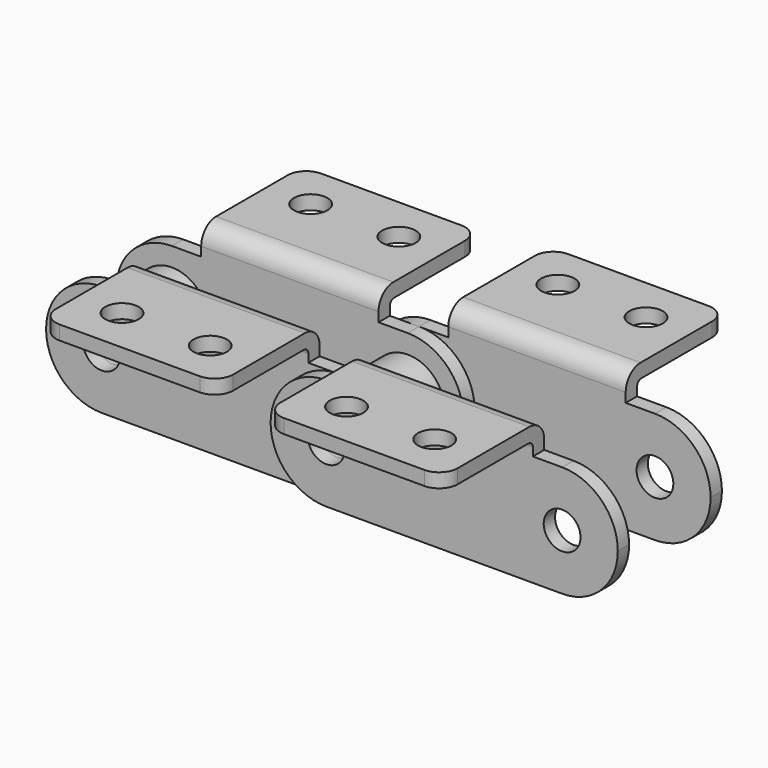
from build123d import *

# Parameters (mm, degrees)
F0_R     = 1.9812
F1_DEPTH = 1.524
F3_DEPTH = 9.5504
F5_D     = 3.6068
F6_R     = 2
F7_R     = 3.9624
F7_R_2   = 1.9812
F8_DEPTH = 7.9248


# Not quite as in the source:
# - a length typed as a fraction of an inch, garbled in the dataset ("3 / 203.2 mm" for 3/8 in), is restored


with BuildPart() as f1:
    # F0 (on Front) → F1 (new body)
    with BuildSketch(Plane.XZ):
        with BuildLine():
            ThreePointArc((-12.7, 5.9944), (-8.4613191109, 4.2386808891), (-6.7056, 0))
            ThreePointArc((-6.7056, 0), (-8.4613191109, -4.2386808891), (-12.7, -5.9944))
            Line((-12.7, -5.9944), (12.7, -5.9944))
            ThreePointArc((12.7, -5.9944), (6.7056, 0), (12.7, 5.9944))
            Line((12.7, 5.9944), (-12.7, 5.9944))
        make_face()
        with BuildLine():
            ThreePointArc((-12.7, -5.9944), (-8.4613191109, -4.2386808891), (-6.7056, 0))
            ThreePointArc((-6.7056, 0), (-8.4613191109, 4.2386808891), (-12.7, 5.9944))
            ThreePointArc((-12.7, 5.9944), (-18.6944, 0), (-12.7, -5.9944))
        make_face()
        with Locations((-12.7, 0)):
            Circle(F0_R, mode=Mode.SUBTRACT)
        with BuildLine():
            ThreePointArc((18.6944, 0), (16.9386808891, 4.2386808891), (12.7, 5.9944))
            ThreePointArc((12.7, 5.9944), (6.7056, 0), (12.7, -5.9944))
            ThreePointArc((12.7, -5.9944), (16.9386808891, -4.2386808891), (18.6944, 0))
        make_face()
        with Locations((12.7, 0)):
            Circle(F0_R, mode=Mode.SUBTRACT)
    extrude(amount=F1_DEPTH)

    # F2 (on Right) → F3 (join, symmetric)
    with BuildSketch(Plane.YZ):
        with BuildLine():
            Line((-1.524, 5.9944), (0, 5.9944))
            Line((0, 5.9944), (0, 6.9944))
            ThreePointArc((0, 6.9944), (-0.5857864376, 8.4086135624), (-2, 8.9944))
            Line((-2, 8.9944), (-13.6398, 8.9944))
            Line((-13.6398, 8.9944), (-13.6398, 7.4704))
            Line((-13.6398, 7.4704), (-2.124, 7.4704))
            ThreePointArc((-2.124, 7.4704), (-1.6997359313, 7.2946640687), (-1.524, 6.8704))
            Line((-1.524, 6.8704), (-1.524, 5.9944))
        make_face()
    extrude(amount=F3_DEPTH, both=True)

    # F5 (through all)
    with Locations(Plane.XY.offset(8.9944)):
        with Locations((-4.7498, -8.7376), (4.7498, -8.7376)):
            Hole(F5_D / 2)

    # F6
    f6_edges = [f1.edges().sort_by_distance(p)[0] for p in [
        (9.5504, -13.6398, 8.2324),
        (-9.5504, -13.6398, 8.2324),
    ]]
    fillet(f6_edges, radius=F6_R)


with BuildPart() as f8:
    # F7 (on Front) → F8 (new body)
    with BuildSketch(Plane.XZ):
        with Locations((-12.7, 0)):
            Circle(F7_R)
        with Locations((-12.7, 0)):
            Circle(F7_R_2, mode=Mode.SUBTRACT)
    extrude(amount=-F8_DEPTH)


with BuildPart() as f8b:
    # F7 (on Front) → F8, piece 2 (new body)
    with BuildSketch(Plane.XZ):
        with Locations((12.7, 0)):
            Circle(F7_R)
        with Locations((12.7, 0)):
            Circle(F7_R_2, mode=Mode.SUBTRACT)
    extrude(amount=-F8_DEPTH)


with BuildPart() as f10_1:
    # F10: instance of F1
    add(f1.part.mirror(Plane.XZ.offset(-3.9624)))


with BuildPart() as f11_1:
    # F11: copy of F1
    add(f1.part.moved(Location((25.4, -1.524, 0))))


with BuildPart() as f12_1:
    # F12: copy of F10_1
    add(f10_1.part.moved(Location((25.4, 1.524, 0))))


solid = Compound([f1.part, f8.part, f8b.part, f10_1.part, f11_1.part, f12_1.part])
